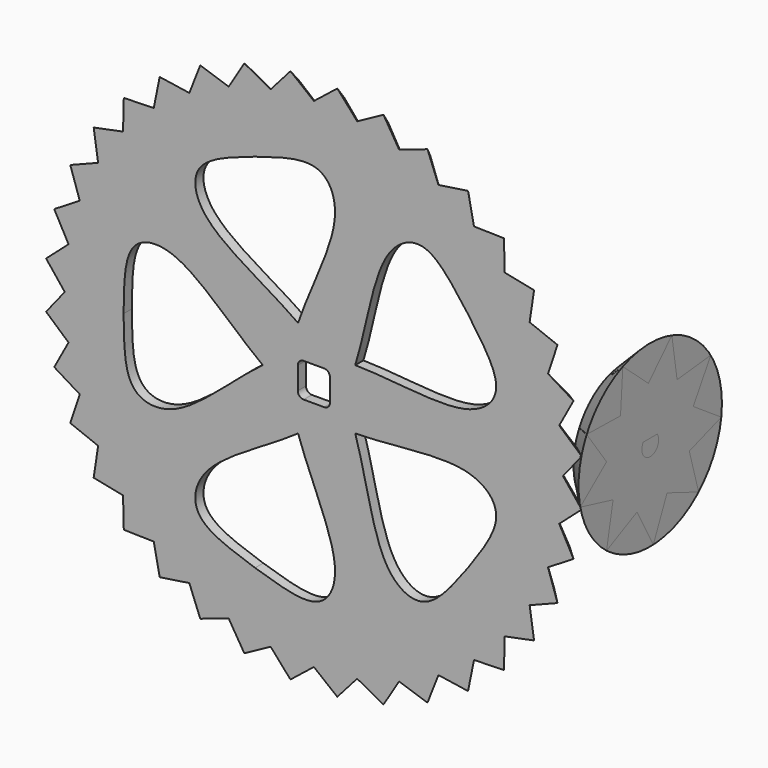
from build123d import *

# Parameters (mm, degrees)
F4_R      = 25
F5_DEPTH  = 10
F5_TAPER  = -45
F11_DEPTH = 10
F13_DEPTH = 7
F14_W     = 12.5930963145
F14_H     = 13.32
F15_DEPTH = 4
F16_R     = 2.3
F18_DEPTH = 4
F19_R     = 1.6
F20_DEPTH = 7.5
F23_DEPTH = 1.5


# Not quite as in the source:
# - ends of sketch curves that miss each other by under 0.0002 mm in the source are joined


with BuildPart() as f3:
    # F1 (on Front) → F3 section 0
    with BuildSketch(Plane.XZ):
        Polygon((-99.6194698092, -8.7155742748), (-90.9038955344, -16.0288094342), (-96.5925826289, -25.8819045103), (-86.7394875529, -31.5705916048), (-90.6307787037, -42.2618261741), (-79.9395441343, -46.1531173249), (-81.9152044289, -57.3576436351), (-70.7106781187, -59.3333039297), (-70.7106781187, -70.7106781187), (-59.3333039297, -70.7106781187), (-57.3576436351, -81.9152044289), (-46.1531173249, -79.9395441343), (-42.2618261741, -90.6307787037), (-31.5705916048, -86.7394875529), (-25.8819045103, -96.5925826289), (-16.0288094342, -90.9038955344), (-8.7155742748, -99.6194698092), (0, -92.3062346497), (8.7155742748, -99.6194698092), (16.0288094342, -90.9038955344), (25.8819045103, -96.5925826289), (31.5705916047, -86.7394875529), (42.2618261741, -90.6307787037), (46.1531173249, -79.9395441343), (57.3576436351, -81.9152044289), (59.3333039297, -70.7106781187), (70.7106781187, -70.7106781187), (70.7106781187, -59.3333039297), (81.9152044289, -57.3576436351), (79.9395441343, -46.1531173249), (90.6307787037, -42.2618261741), (86.7394875529, -31.5705916048), (96.5925826289, -25.8819045103), (90.9038955344, -16.0288094342), (99.6194698092, -8.7155742748), (92.3062346497, 0), (99.6194698092, 8.7155742748), (90.9038955344, 16.0288094342), (96.5925826289, 25.8819045103), (86.7394875529, 31.5705916048), (90.6307787037, 42.2618261741), (79.9395441343, 46.1531173249), (81.9152044289, 57.3576436351), (70.7106781187, 59.3333039297), (70.7106781187, 70.7106781187), (59.3333039297, 70.7106781187), (57.3576436351, 81.9152044289), (46.1531173249, 79.9395441343), (42.2618261741, 90.6307787037), (31.5705916048, 86.7394875529), (25.8819045103, 96.5925826289), (16.0288094342, 90.9038955344), (8.7155742748, 99.6194698092), (0, 92.3062346497), (-8.7155742748, 99.6194698092), (-16.0288094342, 90.9038955344), (-25.8819045103, 96.5925826289), (-31.5705916048, 86.7394875529), (-42.2618261741, 90.6307787037), (-46.1531173249, 79.9395441343), (-57.3576436351, 81.9152044289), (-59.3333039297, 70.7106781187), (-70.7106781187, 70.7106781187), (-70.7106781187, 59.3333039297), (-81.9152044289, 57.3576436351), (-79.9395441343, 46.1531173249), (-90.6307787037, 42.2618261741), (-86.7394875529, 31.5705916048), (-96.5925826289, 25.8819045103), (-90.9038955344, 16.0288094342), (-99.6194698092, 8.7155742748), (-92.3062346497, 0), align=None)
    # F2 (on offset) → F3 section 1
    with BuildSketch(Plane.XZ.offset(4)):
        Polygon((-44.3749174828, 95.1623176388), (-48.653115, 84.2696671265), (-60.2255258169, 86.0109646503), (-62.5472389893, 74.5408967724), (-74.2462120246, 74.2462120246), (-74.5408967724, 62.5472389893), (-86.0109646503, 60.2255258169), (-84.2696671265, 48.653115), (-95.1623176388, 44.3749174828), (-91.4379462875, 33.2806907311), (-101.4222117604, 27.1759997358), (-95.8279297204, 16.8970495151), (-104.6004432996, 9.1513529885), (-97.30623, 0), (-104.6004432996, -9.1513529885), (-95.8279297204, -16.8970495151), (-101.4222117604, -27.1759997358), (-91.4379462875, -33.2806907311), (-95.1623176388, -44.3749174828), (-84.2696671265, -48.653115), (-86.0109646503, -60.2255258169), (-74.5408967724, -62.5472389893), (-74.2462120246, -74.2462120246), (-62.5472389893, -74.5408967724), (-60.2255258169, -86.0109646503), (-48.653115, -84.2696671265), (-44.3749174828, -95.1623176388), (-33.2806907311, -91.4379462875), (-27.1759997358, -101.4222117604), (-16.8970495151, -95.8279297204), (-9.1513529885, -104.6004432996), (0, -97.30623), (9.1513529885, -104.6004432996), (16.8970495151, -95.8279297204), (27.1759997358, -101.4222117604), (33.2806907311, -91.4379462875), (44.3749174828, -95.1623176388), (48.653115, -84.2696671265), (60.2255258169, -86.0109646503), (62.5472389893, -74.5408967724), (74.2462120246, -74.2462120246), (74.5408967724, -62.5472389893), (86.0109646503, -60.2255258169), (84.2696671265, -48.653115), (95.1623176388, -44.3749174828), (91.4379462875, -33.2806907311), (101.4222117604, -27.1759997358), (95.8279297204, -16.8970495151), (104.6004432996, -9.1513529885), (97.30623, 0), (104.6004432996, 9.1513529885), (95.8279297204, 16.8970495151), (101.4222117604, 27.1759997358), (91.4379462875, 33.2806907311), (95.1623176388, 44.3749174828), (84.2696671265, 48.653115), (86.0109646503, 60.2255258169), (74.5408967724, 62.5472389893), (74.2462120246, 74.2462120246), (62.5472389893, 74.5408967724), (60.2255258169, 86.0109646503), (48.653115, 84.2696671265), (44.3749174828, 95.1623176388), (33.2806907311, 91.4379462875), (27.1759997358, 101.4222117604), (16.8970495151, 95.8279297204), (9.1513529885, 104.6004432996), (0, 97.30623), (-9.1513529885, 104.6004432996), (-16.8970495151, 95.8279297204), (-27.1759997358, 101.4222117604), (-33.2806907311, 91.4379462875), align=None)
    loft()

    # F14 (on face) → F15 (cut, through all)
    with BuildSketch(Plane.XZ.offset(4)):
        Rectangle(F14_W, F14_H)
    extrude(amount=-F15_DEPTH, mode=Mode.SUBTRACT)

    # F16
    f16_edges = [f3.edges().sort_by_distance(p)[0] for p in [
        (6.296548, -2, 6.66),
        (-6.296548, -2, 6.66),
        (-6.296548, -2, -6.66),
        (6.296548, -2, -6.66),
    ]]
    fillet(f16_edges, radius=F16_R)

    # F17 (on face) → F18 (cut, through all)
    with BuildSketch(Plane.XZ):
        with BuildLine():
            add(Edge.make_bspline(
                [(60.1382432509, -43.6929912813), (54.0321668924, -51.8091729871), (44.1122228529, -65.7714923569), (23.9113818977, -54.5767028499), (20.9545476799, -27.26973187), (16.1557617381, -11.737847975)],
                knots=[0, 0, 0, 0, 0.3209664482, 0.5727556843, 1, 1, 1, 1], degree=3))
            add(Edge.make_bspline(
                [(60.1382432509, -43.6929912813), (65.9703093859, -35.377729495), (76.1838329137, -21.6287081088), (59.2945522487, -5.8759468899), (32.4103675351, -11.5021485371), (16.1557617381, -11.737847975)],
                knots=[0, 0, 0, 0, 0.3209664482, 0.5727556843, 1, 1, 1, 1], degree=3))
        make_face()
        with BuildLine():
            add(Edge.make_bspline(
                [(60.1382432509, 43.6929912813), (65.9703093859, 35.377729495), (76.1838329137, 21.6287081088), (59.2945522487, 5.8759468899), (32.4103675351, 11.5021485371), (16.1557617381, 11.737847975)],
                knots=[0, 0, 0, 0, 0.3209664482, 0.5727556843, 1, 1, 1, 1], degree=3))
            add(Edge.make_bspline(
                [(60.1382432509, 43.6929912813), (54.0321668924, 51.8091729871), (44.1122228529, 65.7714923569), (23.9113818977, 54.5767028499), (20.9545476799, 27.26973187), (16.1557617381, 11.737847975)],
                knots=[0, 0, 0, 0, 0.3209664482, 0.5727556843, 1, 1, 1, 1], degree=3))
        make_face()
        with BuildLine():
            add(Edge.make_bspline(
                [(-22.9707648981, 70.6967449634), (-13.2602734435, 73.6738122598), (2.971975281, 79.1387691009), (12.7346667397, 58.2082377439), (-0.9238389554, 34.3784506096), (-6.1709518698, 18.9922369784)],
                knots=[0, 0, 0, 0, 0.3209664482, 0.5727556843, 1, 1, 1, 1], degree=3))
            add(Edge.make_bspline(
                [(-22.9707648981, 70.6967449634), (-32.5765937606, 67.3975593301), (-48.9209798713, 62.2777258762), (-44.5165055179, 39.606204245), (-19.45974485, 28.3557696969), (-6.1709518698, 18.9922369784)],
                knots=[0, 0, 0, 0, 0.3209664482, 0.5727556843, 1, 1, 1, 1], degree=3))
        make_face()
        with BuildLine():
            add(Edge.make_bspline(
                [(-74.3349567056, 0), (-74.1656090741, 10.1551905624), (-74.3470511763, 27.2817410233), (-51.4240953682, 30.0987224611), (-32.9813314096, 9.7449024201), (-19.9696197366, 0)],
                knots=[0, 0, 0, 0, 0.3209664482, 0.5727556843, 1, 1, 1, 1], degree=3))
            add(Edge.make_bspline(
                [(-74.3349567056, 0), (-74.1656090741, -10.1551905624), (-74.3470511763, -27.2817410233), (-51.4240953682, -30.0987224611), (-32.9813314096, -9.7449024201), (-19.9696197366, 0)],
                knots=[0, 0, 0, 0, 0.3209664482, 0.5727556843, 1, 1, 1, 1], degree=3))
        make_face()
        with BuildLine():
            add(Edge.make_bspline(
                [(-22.9707648981, -70.6967449634), (-32.5765937606, -67.3975593301), (-48.9209798713, -62.2777258762), (-44.5165055179, -39.606204245), (-19.45974485, -28.3557696969), (-6.1709518698, -18.9922369784)],
                knots=[0, 0, 0, 0, 0.3209664482, 0.5727556843, 1, 1, 1, 1], degree=3))
            add(Edge.make_bspline(
                [(-22.9707648981, -70.6967449634), (-13.2602734435, -73.6738122598), (2.971975281, -79.1387691009), (12.7346667397, -58.2082377439), (-0.9238389554, -34.3784506096), (-6.1709518698, -18.9922369784)],
                knots=[0, 0, 0, 0, 0.3209664482, 0.5727556843, 1, 1, 1, 1], degree=3))
        make_face()
    extrude(amount=F18_DEPTH, mode=Mode.SUBTRACT)


with BuildPart() as f5:
    # F4 (on Right) → F5 (new body)
    with BuildSketch(Plane.YZ):
        with Locations((42.328465167, 0)):
            Circle(F4_R)
    extrude(amount=F5_DEPTH, taper=F5_TAPER)


with BuildPart() as f5_1:
    # F6: moved
    add(f5.part.moved(Location((95.2, -13.6, 0))))


with BuildPart() as f9:
    # F8 (on face) → F9 section 0
    with BuildSketch(Plane.YZ.offset(105.2)):
        Polygon((49.7289206247, 4.6392224517), (58.2612144492, 18.7834160853), (41.8337126628, 17.0526831455), (39.2781165174, 33.3722168335), (27.806413749, 21.4870038761), (15.3587194725, 32.3457864345), (14.2105529411, 15.8673166916), (-2.3048249739, 16.1844030794), (7.4077846123, 2.8231356815), (-5.4475480667, -7.5498423462), (10.581199668, -11.5420218896), (7.4010652566, -27.7514326308), (22.2459219351, -20.5065391433), (30.2290060255, -34.9678191647), (36.9438982258, -19.875818827), (52.3548270502, -25.8223744873), (47.7977820839, -9.9449819865), (63.4256107718, -4.5943538037), align=None)
    # F7 (on face) → F9 section 1
    with BuildSketch(Plane(origin=(95.2, 0, 0), x_dir=(0, -1, 0), z_dir=(-1, 0, 0))):
        Polygon((-28.0878709009, 14.9280736511), (-36.2639304173, 23.8372977382), (-37.8333222686, 11.8473339239), (-49.8232860828, 13.4167257752), (-43.3185098092, 3.2230949853), (-53.512140599, -3.2816812883), (-41.9768533114, -6.9092659176), (-45.6044379407, -18.4445532052), (-34.4361287614, -13.8087045098), (-29.800280066, -24.977013689), (-24.224724982, -14.2468967952), (-13.4946080881, -19.8224518791), (-16.1206712886, -8.0188077335), (-4.3170271429, -5.392744533), (-13.9159444709, 1.9613705858), (-6.5618293521, 11.5602879138), (-18.6421607097, 11.0238018098), (-19.1786468138, 23.1041331675), align=None)
    loft()

    # F10 (on face) → F11 (cut, through all)
    with BuildSketch(Plane.YZ.offset(105.2)):
        with BuildLine():
            Line((28.728465167, 2.3), (25.3343526173, 2.3))
            ThreePointArc((25.3343526173, 2.3), (28.728465167, -4.1), (32.1225777167, 2.3))
            Line((32.1225777167, 2.3), (28.728465167, 2.3))
        make_face()
    extrude(amount=-F11_DEPTH, mode=Mode.SUBTRACT)

    # F12 (on face) → F13 (join)
    with BuildSketch(Plane(origin=(95.2, 0, 0), x_dir=(0, -1, 0), z_dir=(-1, 0, 0))):
        with BuildLine():
            Line((-23.4343526173, 9.8), (-28.728465167, 9.8))
            Line((-28.728465167, 9.8), (-34.0225777167, 9.8))
            Line((-34.0225777167, 9.8), (-34.0225777167, 8.9))
            Line((-34.0225777167, 8.9), (-34.0225777167, 4.7310011954))
            ThreePointArc((-34.0225777167, 4.7310011954), (-28.728465167, -7.1), (-23.4343526173, 4.7310011954))
            Line((-23.4343526173, 4.7310011954), (-23.4343526173, 8.9))
            Line((-23.4343526173, 8.9), (-23.4343526173, 9.8))
        make_face()
        with BuildLine():
            Line((-28.728465167, 2.3), (-25.3343526173, 2.3))
            Line((-25.3343526173, 2.3), (-25.2142084888, 2.3))
            ThreePointArc((-25.2142084888, 2.3), (-28.728465167, -4.2), (-32.2427218451, 2.3))
            Line((-32.2427218451, 2.3), (-32.1225777167, 2.3))
            Line((-32.1225777167, 2.3), (-28.728465167, 2.3))
        make_face(mode=Mode.SUBTRACT)
    extrude(amount=F13_DEPTH)

    # F19 (on face) → F20 (cut, through all)
    with BuildSketch(Plane.XY.offset(9.8)):
        with Locations((91.7, 28.728465167)):
            Circle(F19_R)
    extrude(amount=-F20_DEPTH, mode=Mode.SUBTRACT)

    # F22 (on offset) → F23 (cut, symmetric)
    with BuildSketch(Plane.XY.offset(6.05)):
        Polygon((90.402888234, 28.728465167), (91.7, 28.728465167), (95.1971168681, 28.728465167), (95.1971168681, 30.9784666398), (91.3000025511, 33.2284666398), (90.402888234, 33.2284666398), align=None)
        Polygon((95.1971168681, 28.728465167), (91.7, 28.728465167), (90.402888234, 28.728465167), (90.402888234, 24.228465167), (91.3000025511, 24.2284666398), (95.1971168681, 26.4784666398), align=None)
        Polygon((90.402888234, 24.228465167), (90.402888234, 28.728465167), (87.402888234, 28.728465167), (87.402888234, 26.4784666398), (87.402888234, 24.2284666398), align=None)
        Polygon((87.402888234, 28.728465167), (90.402888234, 28.728465167), (90.402888234, 33.228465167), (87.402888234, 33.2284666398), (87.402888234, 30.9784666398), align=None)
        Polygon((84.402888234, 28.728465167), (87.402888234, 28.728465167), (87.402888234, 30.9784666398), (87.402888234, 33.2284666398), (84.402888234, 33.228465167), align=None)
        Polygon((87.402888234, 26.4784666398), (87.402888234, 28.728465167), (84.402888234, 28.728465167), (84.402888234, 24.228465167), (87.402888234, 24.228465167), align=None)
    extrude(amount=F23_DEPTH, both=True, mode=Mode.SUBTRACT)


solid = Compound([f3.part, f5_1.part, f9.part])
